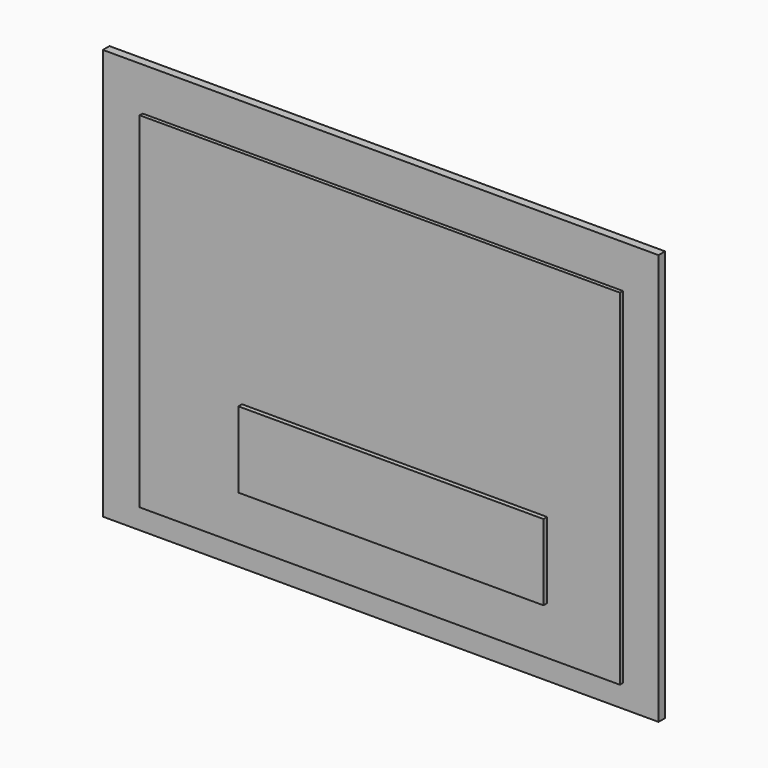
from build123d import *

# Parameters (mm, degrees)
F2_W     = 185.8412176371
F2_H     = 137.4446004629
F3_DEPTH = 2.76111
F5_W     = 160.6390327215
F5_H     = 115.4496371746
F6_DEPTH = 1.25079
F7_W     = 102.049253881
F7_H     = 25.4090260714
F8_DEPTH = 1.51544


# Not quite as in the source:
# - the program builds the solid bodies; features that only make, move or delete a surface that nothing else refers to are left out


with BuildPart() as f3:
    # F2 (on Front) → F3 (new body)
    with BuildSketch(Plane.XZ):
        with Locations((-17.6170766354, -5.8681294322)):
            Rectangle(F2_W, F2_H)
    extrude(amount=-F3_DEPTH)


with BuildPart() as f6:
    # F5 (on face) → F6 (new body)
    with BuildSketch(Plane.XZ):
        with Locations((-16.9224664569, -9.2854946852)):
            Rectangle(F5_W, F5_H)
    extrude(amount=F6_DEPTH)


with BuildPart() as f8:
    # F7 (on face) → F8 (new body)
    with BuildSketch(Plane.XZ.offset(1.25079)):
        with Locations((-11.9856484234, -38.2217699662)):
            Rectangle(F7_W, F7_H)
    extrude(amount=F8_DEPTH)


solid = Compound([f3.part, f6.part, f8.part])
